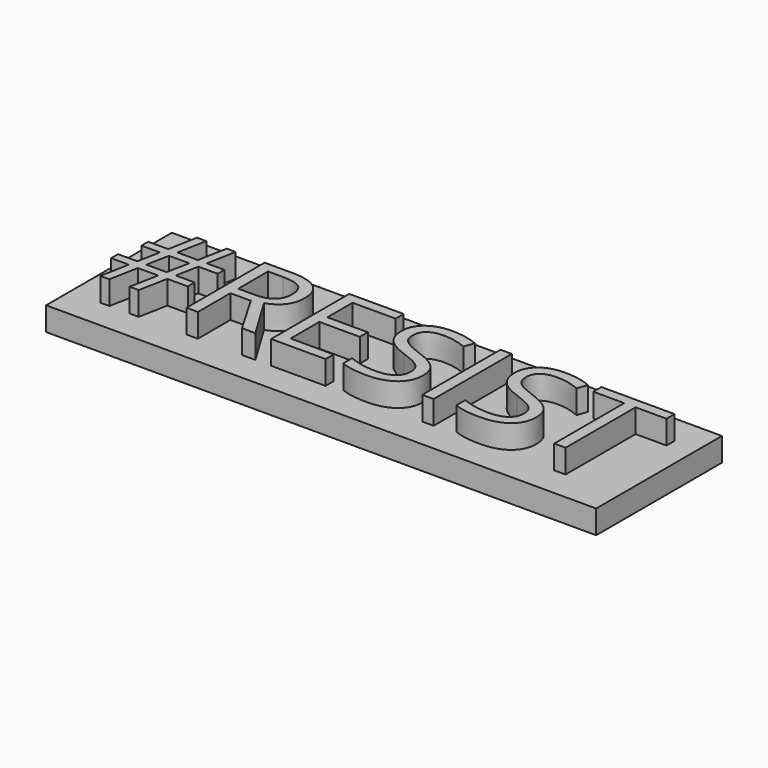
from build123d import *

# Parameters (mm, degrees)
F0_W         = 35
F0_H         = 10
F1_DEPTH     = 1.5
F2_TEXT_SIZE = 8.7033473058
F3_DEPTH     = 3


# Not quite as in the source:
# - Text() gives the source's letters only with a copy of the font that has no kerning and outlines rounded to 1/6400 em; it was checked with that copy


with BuildPart() as f1:
    # F0 (on Top) → F1 (new body)
    with BuildSketch(Plane.XY):
        Rectangle(F0_W, F0_H)
    extrude(amount=F1_DEPTH)

    # F2 (on Top) → F3 (join)
    with BuildSketch(Plane.XY):
        with Locations((-16.5601580963, -3.0963899079)):
            Text('#RESIST', F2_TEXT_SIZE, font='Open Sans', text_align=(TextAlign.LEFT, TextAlign.BOTTOM))
    extrude(amount=F3_DEPTH)


solid = f1.part
